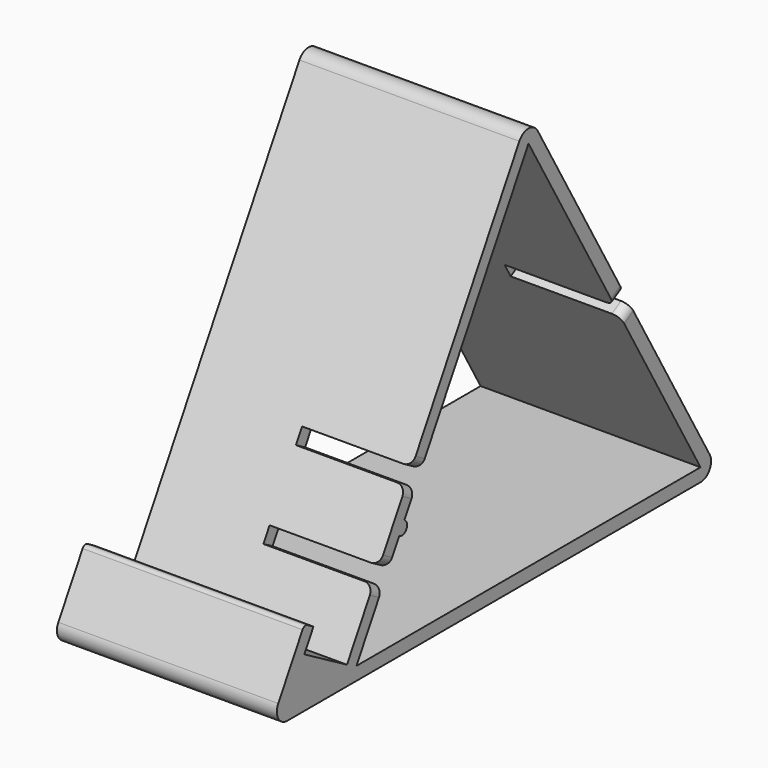
from build123d import *

# Parameters (mm, degrees)
F1_DEPTH  = 50
F2_T      = 3
F4_DEPTH  = 50
F5_W      = 25
F5_H      = 3.5
F6_DEPTH  = 3
F7_W      = 25
F7_H      = 3.5
F8_DEPTH  = 3
F9_R      = 2
F10_R     = 1.5
F11_DEPTH = 50
F12_W     = 25
F12_H     = 3.5
F13_DEPTH = 10
F14_R     = 2


# Not quite as in the source:
# - a shell that OpenCascade refuses in one call is made with other operations: the cavity is built on its own and cut out


with BuildPart() as f1:
    # F0 (on Right) → F1 (new body)
    with BuildSketch(Plane.YZ):
        with BuildLine():
            Line((-2.5980762114, 57.9554029985), (-54.0879656003, -31.2277014993))
            Line((-54.0879656003, -31.2277014993), (48.8918131776, -31.2277014993))
            ThreePointArc((48.8918131776, -31.2277014993), (51.4898893889, -29.7277014993), (51.4898893889, -26.7277014993))
            Line((51.4898893889, -26.7277014993), (2.5980762114, 57.9554029985))
            ThreePointArc((2.5980762114, 57.9554029985), (0, 59.4554029985), (-2.5980762114, 57.9554029985))
        make_face()
    extrude(amount=F1_DEPTH)

    # F2: shell of thickness 3, made by hand


with BuildPart() as f2_core1:
    # F2_t2: copy of F1
    add(f1.part)

    # the walls: a layer under each face that stays
    f2_faces = [f2_core1.faces().sort_by_distance(p)[0] for p in [
        (25, -28.3430209058, 13.3638507496),
        (25, -2.5980762114, -31.2277014993),
        (25, 27.0439828001, 15.6138507496),
    ]]
    thicken(f2_faces, amount=-F2_T, mode=Mode.SUBTRACT)


with BuildPart() as f1_1:
    add(f1.part)

    # what is left inside the walls is the cavity
    f2_cavity = [f2_core1.part.solids().sort_by_distance(p)[0] for p in [
        (33.333333, -24.419926, 14.098851),
    ]]
    add(f2_cavity, mode=Mode.SUBTRACT)

    # F3 (on Right) → F4 (join)
    with BuildSketch(Plane.YZ):
        with BuildLine():
            Line((-54.0879656003, -31.2277014993), (-51.5879656003, -26.8975744803))
            Line((-51.5879656003, -26.8975744803), (-63.7123212533, -19.8975744803))
            Line((-63.7123212533, -19.8975744803), (-61.1142450419, -15.3975744803))
            Line((-61.1142450419, -15.3975744803), (-62.8462958495, -14.3975744803))
            ThreePointArc((-62.8462958495, -14.3975744803), (-63.6051148946, -14.2976740578), (-64.2123212533, -14.7635998841))
            Line((-64.2123212533, -14.7635998841), (-71.1197985414, -26.7277014993))
            ThreePointArc((-71.1197985414, -26.7277014993), (-71.1197985414, -29.7277014993), (-68.52172233, -31.2277014993))
            Line((-68.52172233, -31.2277014993), (-54.0879656003, -31.2277014993))
        make_face()
    extrude(amount=F4_DEPTH)

    # F5 (on face) → F6 (cut, through all)
    with BuildSketch(Plane(origin=(0, -27.0439828002, 15.6138507496), x_dir=(1, 0, 0), z_dir=(0, -0.8660254038, 0.5))):
        with Locations((37.5, -32.3379656003)):
            Rectangle(F5_W, F5_H)
    extrude(amount=-F6_DEPTH, mode=Mode.SUBTRACT)

    # F7 (on face) → F8 (cut, through all)
    with BuildSketch(Plane(origin=(0, -27.0439828002, 15.6138507496), x_dir=(1, 0, 0), z_dir=(0, -0.8660254038, 0.5))):
        with Locations((37.5, -13.8379656003)):
            Rectangle(F7_W, F7_H)
    extrude(amount=-F8_DEPTH, mode=Mode.SUBTRACT)

    # F9
    f9_edges = [f1_1.edges().sort_by_distance(p)[0] for p in [
        (50, -31.788927, 4.395365),
        (50, -33.538927, 1.364277),
        (50, -41.038927, -11.626105),
        (50, -42.788927, -14.657193),
    ]]
    fillet(f9_edges, radius=F9_R)

    # F10 (on Right) → F11 (join)
    with BuildSketch(Plane.YZ):
        with Locations((-35.9918131776, -5.8842460816)):
            Circle(F10_R)
    extrude(amount=F11_DEPTH)

    # F12 (on face) → F13 (cut)
    with BuildSketch(Plane(origin=(0, 27.0439828001, 15.6138507496), x_dir=(-1, 0, 0), z_dir=(0, 0.8660254038, 0.5))):
        with Locations((-37.5, -1.75)):
            Rectangle(F12_W, F12_H)
    extrude(amount=-F13_DEPTH, mode=Mode.SUBTRACT)

    # F14
    f14_edges = [f1_1.edges().sort_by_distance(p)[0] for p in [
        (50, 27.494945, 11.832762),
        (50, 25.744945, 14.863851),
    ]]
    fillet(f14_edges, radius=F14_R)


solid = f1_1.part
